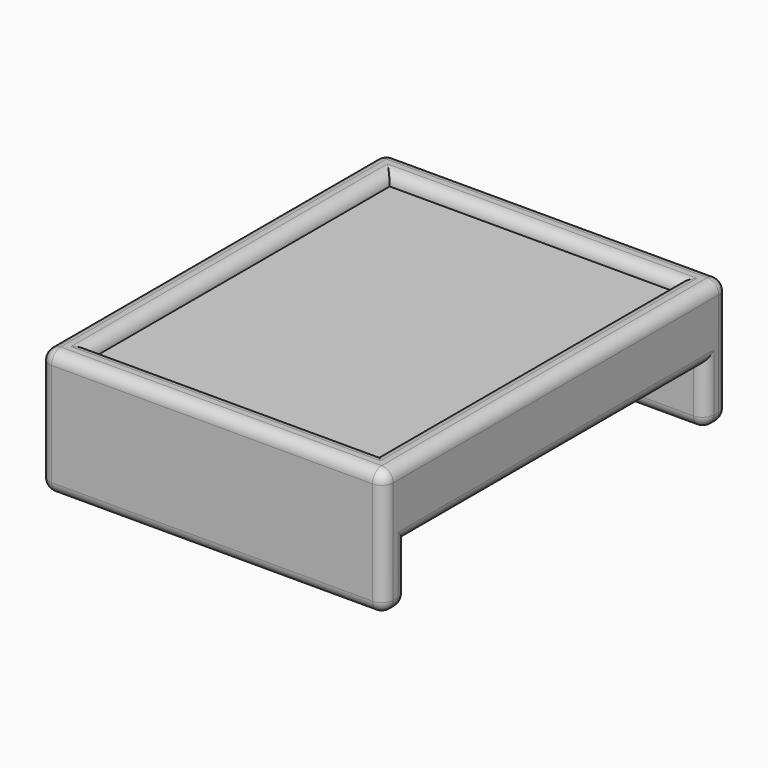
from build123d import *

# Parameters (mm, degrees)
F0_W     = 25
F0_H     = 32.5
F0_W_2   = 2.5
F1_DEPTH = 5
F2_DEPTH = 6
F3_DEPTH = 5
F4_R     = 0.99999


# Not quite as in the source:
# - a fillet or chamfer is up to 0.001 mm smaller than in the source, because OpenCascade refuses the exact size


with BuildPart() as f1:
    # F0 (on Top) → F1 (new body)
    with BuildSketch(Plane.XY):
        Rectangle(F0_W, F0_H)
        Polygon((-15, 16.25), (-12.5, 16.25), (12.5, 16.25), (15, 16.25), (15, 18.75), (-15, 18.75), align=None)
        with Locations((-13.75, 0)):
            Rectangle(F0_W_2, F0_H)
        Polygon((12.5, -16.25), (-12.5, -16.25), (-15, -16.25), (-15, -18.75), (15, -18.75), (15, -16.25), align=None)
        with Locations((13.75, 0)):
            Rectangle(F0_W_2, F0_H)
    extrude(amount=F1_DEPTH)

    # F0 (on Top) → F2 (join)
    with BuildSketch(Plane.XY):
        Polygon((-15, 16.25), (-12.5, 16.25), (12.5, 16.25), (15, 16.25), (15, 18.75), (-15, 18.75), align=None)
        with Locations((-13.75, 0)):
            Rectangle(F0_W_2, F0_H)
        Polygon((12.5, -16.25), (-12.5, -16.25), (-15, -16.25), (-15, -18.75), (15, -18.75), (15, -16.25), align=None)
        with Locations((13.75, 0)):
            Rectangle(F0_W_2, F0_H)
    extrude(amount=F2_DEPTH)

    # F0 (on Top) → F3 (join)
    with BuildSketch(Plane.XY):
        Polygon((12.5, -16.25), (-12.5, -16.25), (-15, -16.25), (-15, -18.75), (15, -18.75), (15, -16.25), align=None)
        Polygon((-15, 16.25), (-12.5, 16.25), (12.5, 16.25), (15, 16.25), (15, 18.75), (-15, 18.75), align=None)
    extrude(amount=-F3_DEPTH)

    # F4 (radius 1 in the source; OpenCascade refuses exactly that, so slightly less here)
    f4_edges = [f1.edges().sort_by_distance(p)[0] for p in [
        (0, 16.25, -5),
        (15, 17.5, -5),
        (0, 18.75, -5),
        (-15, 17.5, -5),
        (-15, -17.5, -5),
        (0, -18.75, -5),
        (15, -17.5, -5),
        (0, -16.25, -5),
        (0, 16.25, 6),
        (12.5, 0, 6),
        (0, -16.25, 6),
        (-12.5, 0, 6),
        (0, 18.75, 6),
        (-15, 0, 6),
        (0, -18.75, 6),
        (15, 0, 6),
        (-15, -18.75, 0.5),
        (-15, -16.25, -2.5),
        (-15, 0, 0),
        (-15, 16.25, -2.5),
        (-15, 18.75, 0.5),
        (15, 18.75, 0.5),
        (15, -18.75, 0.5),
        (15, 16.25, -2.5),
        (15, 0, 0),
        (15, -16.25, -2.5),
    ]]
    fillet(f4_edges, radius=F4_R)


solid = f1.part
